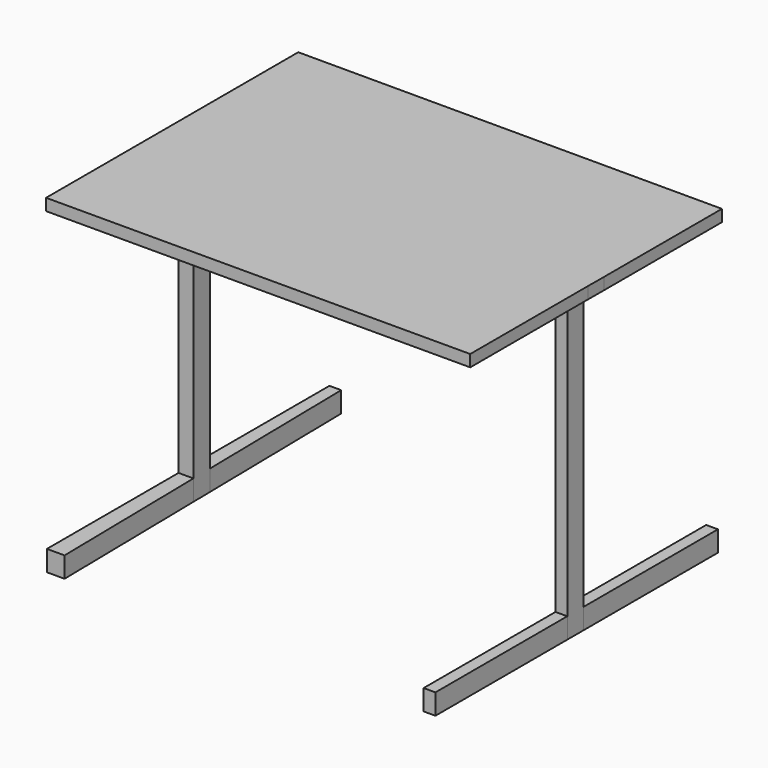
from build123d import *

# Parameters (mm, degrees)
F1_DEPTH = 44.45
F0_W     = 25.4
F0_H     = 355.6
F0_H_2   = 361.95
F2_DEPTH = 660.4
F0_H_3   = 44.45
F3_DEPTH = 44.45
F5_DEPTH = 25.4


with BuildPart() as f1:
    # F0 (on Top) → F1 (new body)
    with BuildSketch(Plane.XY):
        Polygon((-20.4151007465, -385.0066614151), (-52.5996065524, -385.0066614151), (-52.5996065524, -739.9363130581), (-14.4996065524, -739.9363130581), align=None)
    extrude(amount=F1_DEPTH)


with BuildPart() as f1b:
    # F0 (on Top) → F1, piece 2 (new body)
    with BuildSketch(Plane.XY):
        with Locations((772.9003934476, -562.1363130581)):
            Rectangle(F0_W, F0_H)
    extrude(amount=F1_DEPTH)


with BuildPart() as f1c:
    # F0 (on Top) → F1, piece 3 (new body)
    with BuildSketch(Plane.XY):
        with Locations((772.9003934476, -158.9113130581)):
            Rectangle(F0_W, F0_H_2)
    extrude(amount=F1_DEPTH)


with BuildPart() as f1d:
    # F0 (on Top) → F1, piece 4 (new body)
    with BuildSketch(Plane.XY):
        Polygon((-27.1996065524, 22.0636869419), (-52.5996065524, 22.0636869419), (-52.5996065524, -339.8863130581), (-21.1671065524, -339.8863130581), align=None)
    extrude(amount=F1_DEPTH)


with BuildPart() as f2:
    # F0 (on Top) → F2 (new body)
    with BuildSketch(Plane.XY):
        Polygon((-21.1671065524, -339.8863130581), (-52.5996065524, -339.8863130581), (-52.5996065524, -385.0066614151), (-20.4151007465, -385.0066614151), align=None)
    extrude(amount=F2_DEPTH)


with BuildPart() as f2b:
    # F0 (on Top) → F2, piece 2 (new body)
    with BuildSketch(Plane.XY):
        with Locations((772.9003934476, -362.1113130581)):
            Rectangle(F0_W, F0_H_3)
    extrude(amount=F2_DEPTH)

    # F4 (on face) → F5 (join)
    with BuildSketch(Plane.XY.offset(660.4)):
        Polygon((-84.3496065524, -339.8863130581), (-84.3496065524, -385.0066614151), (-84.3496065524, -702.5066614151), (829.7848851204, -701.2691247463), (829.7848851204, -383.7691247463), (830.0107271194, -340.2135372162), (830.0107271194, -22.7135372162), (-84.3496065524, -22.3863130581), align=None)
        Polygon((-20.4151007465, -385.0066614151), (-52.5996065524, -385.0066614151), (-52.5996065524, -339.8863130581), (-21.1671065524, -339.8863130581), align=None, mode=Mode.SUBTRACT)
        Polygon((-52.5996065524, -339.8863130581), (-52.5996065524, -385.0066614151), (-20.4151007465, -385.0066614151), (-21.1671065524, -339.8863130581), align=None)
    extrude(amount=F5_DEPTH)


with BuildPart() as f3:
    # F0 (on Top) → F3 (new body)
    with BuildSketch(Plane.XY):
        Polygon((-27.1996065524, 22.0636869419), (-52.5996065524, 22.0636869419), (-52.5996065524, -339.8863130581), (-21.1671065524, -339.8863130581), align=None)
    extrude(amount=F3_DEPTH)


with BuildPart() as f3b:
    # F0 (on Top) → F3, piece 2 (new body)
    with BuildSketch(Plane.XY):
        Polygon((-20.4151007465, -385.0066614151), (-52.5996065524, -385.0066614151), (-52.5996065524, -739.9363130581), (-14.4996065524, -739.9363130581), align=None)
    extrude(amount=F3_DEPTH)


with BuildPart() as f3c:
    # F0 (on Top) → F3, piece 3 (new body)
    with BuildSketch(Plane.XY):
        with Locations((772.9003934476, -158.9113130581)):
            Rectangle(F0_W, F0_H_2)
    extrude(amount=F3_DEPTH)


with BuildPart() as f3d:
    # F0 (on Top) → F3, piece 4 (new body)
    with BuildSketch(Plane.XY):
        with Locations((772.9003934476, -562.1363130581)):
            Rectangle(F0_W, F0_H)
    extrude(amount=F3_DEPTH)


solid = Compound([f1.part, f1b.part, f1c.part, f1d.part, f2.part, f2b.part, f3.part, f3b.part, f3c.part, f3d.part])
